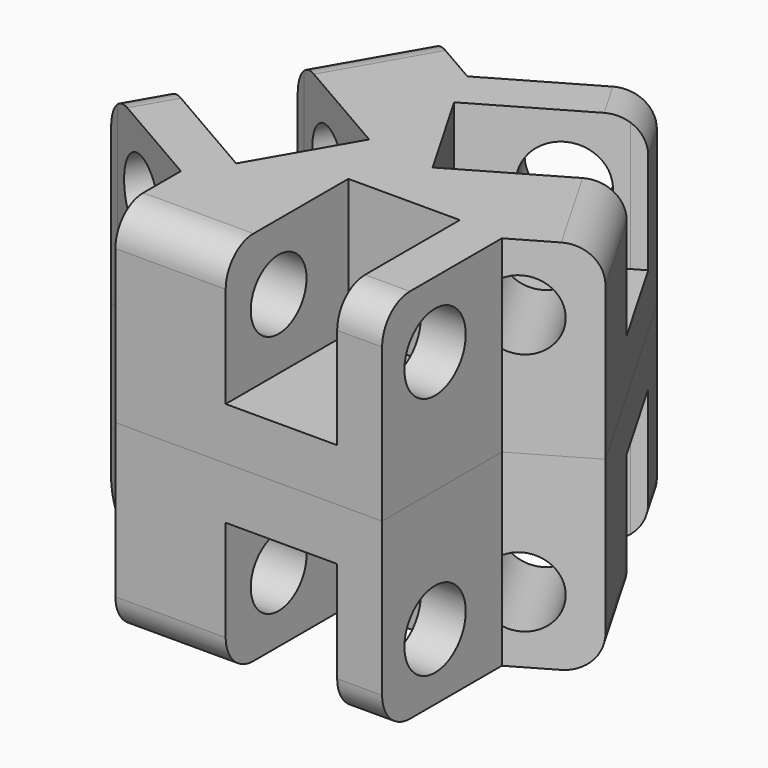
from build123d import *

# Parameters (mm, degrees)
F1_DEPTH  = 5
F2_W      = 3.2
F2_H      = 4
F3_DEPTH  = 3.5
F4_W      = 2.25
F4_H      = 3.897114317
F5_DEPTH  = 5
F6_R      = 1.1
F8_DEPTH  = 1.2895280957
F7_R      = 1.1
F10_DEPTH = 1.2895280957
F9_R      = 1.1
F11_DEPTH = 1.2895280957
F12_R     = 1
F15_REACH = 9.3689552204
F13_R     = 1
F16_REACH = 10.4939552204
F14_R     = 1
F17_REACH = 11.5637192683
F18_DEPTH = 0.4
F19_DEPTH = 0.4
F20_DEPTH = 0.4
F21_DEPTH = 0.4
F22_W     = 1.125
F22_H     = 2.3485571585
F23_DEPTH = 5.4
F24_R     = 1


with BuildPart() as f1:
    # F0 (on Top) → F1 (new body)
    with BuildSketch(Plane.XY):
        Polygon((2.25, 6.367628561), (-2.25, 6.367628561), (-6.6395280957, -1.235257122), (-4.3895280957, -5.132371439), (4.3895280957, -5.132371439), (6.6395280957, -1.235257122), align=None)
    extrude(amount=F1_DEPTH)

    # F2 (on face) → F3 (cut)
    with BuildSketch(Plane.XY.offset(5)):
        with Locations((1.5, -3.132371439)):
            Rectangle(F2_W, F2_H)
        Polygon((4.4947640478, 2.4795831791), (2.8947640478, 5.2508644712), (-0.5693375673, 3.2508644712), (1.0306624327, 0.4795831791), align=None)
        Polygon((-4.3947640478, 2.6527882599), (-5.9947640478, -0.1184930322), (-2.5306624327, -2.1184930322), (-0.9306624327, 0.6527882599), align=None)
    extrude(amount=-F3_DEPTH, mode=Mode.SUBTRACT)

    # F4 (on face) → F5 (cut, through all)
    with BuildSketch(Plane.XY.offset(5)):
        with Locations((5.5145280957, -3.1838142805)):
            Rectangle(F4_W, F4_H)
        Polygon((-1.125, 4.4190714025), (2.25, 6.367628561), (1.125, 8.3161857195), (-2.25, 6.367628561), align=None)
        Polygon((-3.2645280957, -3.1838142805), (-6.6395280957, -1.235257122), (-7.7645280957, -3.1838142805), (-4.3895280957, -5.132371439), align=None)
    extrude(amount=-F5_DEPTH, mode=Mode.SUBTRACT)

    # F6 (on face) → F8 (cut, through all)
    with BuildSketch(Plane(origin=(-2.1947640478, -3.8014428415, 0), x_dir=(0.8660254038, -0.5, 0), z_dir=(-0.5, -0.8660254038, 0))):
        with Locations((-3.632371439, 3.5)):
            Circle(F6_R)
    extrude(amount=-F8_DEPTH, mode=Mode.SUBTRACT)

    # F7 (on face) → F10 (cut, through all)
    with BuildSketch(Plane.YZ.offset(4.3895280957)):
        with Locations((-3.632371439, 3.5)):
            Circle(F7_R)
    extrude(amount=-F10_DEPTH, mode=Mode.SUBTRACT)

    # F9 (on face) → F11 (cut, through all)
    with BuildSketch(Plane(origin=(-2.1947640478, 3.8014428415, 0), x_dir=(-0.8660254038, -0.5, 0), z_dir=(-0.5, 0.8660254038, 0))):
        with Locations((-3.632371439, 3.5)):
            Circle(F9_R)
    extrude(amount=-F11_DEPTH, mode=Mode.SUBTRACT)

    f15_end = Plane(origin=(-3.8270280957, -4.1580928598, 2.5), x_dir=(-0.5, -0.8660254038, 0), z_dir=(-0.8660254038, 0.5, 0))
    # F12 (on face) → F15 (cut, up to a plane its end follows)
    with BuildSketch(Plane.YZ.offset(-0.1)):
        with Locations((-3.632371439, 3.5)):
            Circle(F12_R)
    f15_long = extrude(amount=-F15_REACH, mode=Mode.PRIVATE)
    add(split(f15_long, bisect_by=f15_end, keep=Keep.BOTTOM, mode=Mode.PRIVATE), mode=Mode.SUBTRACT)

    f16_end = Plane(origin=(5.5145280957, -1.235257122, 2.5), x_dir=(0, 0, -1), z_dir=(0, -1, 0))
    # F13 (on face) → F16 (cut, up to a plane its end follows)
    with BuildSketch(Plane(origin=(0.05, -0.0866025404, 0), x_dir=(-0.8660254038, -0.5, 0), z_dir=(-0.5, 0.8660254038, 0))):
        with Locations((-3.632371439, 3.5)):
            Circle(F13_R)
    f16_long = extrude(amount=-F16_REACH, mode=Mode.PRIVATE)
    add(split(f16_long, bisect_by=f16_end, keep=Keep.BOTTOM, mode=Mode.PRIVATE), mode=Mode.SUBTRACT)

    f17_end = Plane(origin=(-1.6875, 5.3933499817, 2.5), x_dir=(-0.5, 0.8660254038, 0), z_dir=(0.8660254038, 0.5, 0))
    # F14 (on face) → F17 (cut, up to a plane its end follows)
    with BuildSketch(Plane(origin=(0.05, 0.0866025404, 0), x_dir=(0.8660254038, -0.5, 0), z_dir=(-0.5, -0.8660254038, 0))):
        with Locations((-3.632371439, 3.5)):
            Circle(F14_R)
    f17_long = extrude(amount=-F17_REACH, mode=Mode.PRIVATE)
    add(split(f17_long, bisect_by=f17_end, keep=Keep.BOTTOM, mode=Mode.PRIVATE), mode=Mode.SUBTRACT)

    # F18 (add): a face of the model
    f18_faces = [f1.faces().sort_by_distance(p)[0] for p in [
        (0, 0, 5),
    ]]
    extrude(f18_faces, amount=F18_DEPTH)

    # F19 (add): a face of the model
    f19_faces = [f1.faces().sort_by_distance(p)[0] for p in [
        (4.7127523056, 2.1020164412, 2.4320117422),
    ]]
    extrude(f19_faces, amount=F19_DEPTH)

    # F20 (add): a face of the model
    f20_faces = [f1.faces().sort_by_distance(p)[0] for p in [
        (-4.1767757901, 3.0303549978, 2.4320117422),
    ]]
    extrude(f20_faces, amount=F20_DEPTH)

    # F21 (add): a face of the model
    f21_faces = [f1.faces().sort_by_distance(p)[0] for p in [
        (-0.5359765155, -5.132371439, 2.4320117422),
    ]]
    extrude(f21_faces, amount=F21_DEPTH)

    # F22 (on face) → F23 (cut, through all)
    with BuildSketch(Plane.XY.offset(5.4)):
        with Locations((-3.8270280957, -4.3580928598)):
            Rectangle(F22_W, F22_H)
        Polygon((6.4234382572, -0.0609785427), (4.3895280957, -1.235257122), (4.9520280957, -2.2095357012), (6.9859382572, -1.035257122), align=None)
        Polygon((-3.1589101615, 5.5933499817), (-1.125, 4.4190714025), (-0.5625, 5.3933499817), (-2.5964101615, 6.567628561), align=None)
    extrude(amount=-F23_DEPTH, mode=Mode.SUBTRACT)

    # F24
    f24_edges = [f1.edges().sort_by_distance(p)[0] for p in [
        (-1.682264, -5.532371, 5.4),
        (3.744764, -5.532371, 5.4),
        (5.632306, 1.309302, 5.4),
        (2.918792, 6.009247, 5.4),
        (-3.950042, 4.223069, 5.4),
        (-6.663556, -0.476875, 5.4),
    ]]
    fillet(f24_edges, radius=F24_R)


with BuildPart() as f25_1:
    # F25: instance of F1
    add(f1.part.mirror(Plane.XY))


solid = Compound([f1.part, f25_1.part])
